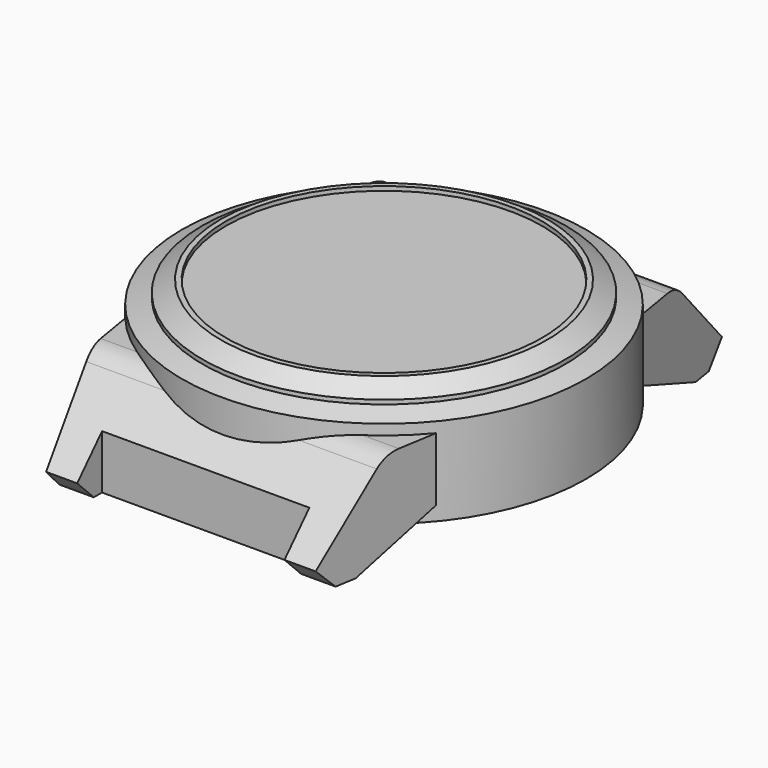
from build123d import *

# Parameters (mm, degrees)
F3_DEPTH         = 15
F5_DEPTH         = 12.601
F5_COPIES2_COUNT = 2
F6_W             = 20
F6_H             = 3
F7_DEPTH         = 12.601


# Not quite as in the source:
# - a pattern or mirror of a feature is missing from the dataset's text; its kind, count and spacing are read off the source's solid


with BuildPart() as f1:
    # F0 (on Front) → F1 (revolve)
    with BuildSketch(Plane.XZ):
        Polygon((-13, 0), (0, 0), (0, 12.2), (-15.25, 12.2), (-15.25, 12.6), (-15.75, 12.6), (-17.5, 11.5), (-17.5, 11.1), (-19.5, 10.5), (-19.5, 2), (-17, 2), align=None)
    revolve(axis=Axis((0, 0, 3.4052523688), (0, 0, -1)))

    # F2 (on Right) → F3 (join, symmetric)
    with BuildSketch(Plane.YZ):
        with BuildLine():
            Line((20.5, 0), (22.5, 0))
            Line((22.5, 0), (24.5, 2))
            Line((24.5, 2), (18.389508899, 8.5469547511))
            ThreePointArc((18.389508899, 8.5469547511), (17.3919884737, 9.2514418269), (16.1963430943, 9.5))
            Line((16.1963430943, 9.5), (11, 9.5))
            Line((11, 9.5), (11, 4))
            Line((11, 4), (20.5, 0))
        make_face()
    f3 = extrude(amount=F3_DEPTH, both=True)

    # F3_copies: F3 across plane
    add(f3.mirror(Plane(origin=(0, 0, 0), x_dir=(0, 0, -1), z_dir=(0, -1, 0))))

    # F4 (on Top) → F5 (cut, through all)
    with BuildSketch(Plane.XY):
        Polygon((-15, 24.5), (-15, 12.4599357944), (-13, 24.5), align=None)
    f5 = extrude(amount=F5_DEPTH, mode=Mode.SUBTRACT)

    # F5_copies: F5 across plane
    add(f5.mirror(Plane(origin=(0, 0, 0), x_dir=(0, 0, 1), z_dir=(1, 0, 0))), mode=Mode.SUBTRACT)

    # F5_copies1: F5 across plane
    add(f5.mirror(Plane(origin=(0, 0, 0), x_dir=(0, 0, -1), z_dir=(0, -1, 0))), mode=Mode.SUBTRACT)

    # F5_copies2: F5 ×2 about axis
    f5_copies2_axis = Axis((0, 0, 0), (0, 0, 1))
    for i in range(1, F5_COPIES2_COUNT):
        add(f5.rotate(f5_copies2_axis, i * 360 / F5_COPIES2_COUNT), mode=Mode.SUBTRACT)

    # F6 (on Top) → F7 (cut, through all)
    with BuildSketch(Plane.XY):
        with Locations((0, 23)):
            Rectangle(F6_W, F6_H)
    f7 = extrude(amount=F7_DEPTH, mode=Mode.SUBTRACT)

    # F7_copies: F7 across plane
    add(f7.mirror(Plane(origin=(0, 0, 0), x_dir=(0, 0, -1), z_dir=(0, -1, 0))), mode=Mode.SUBTRACT)


solid = f1.part
